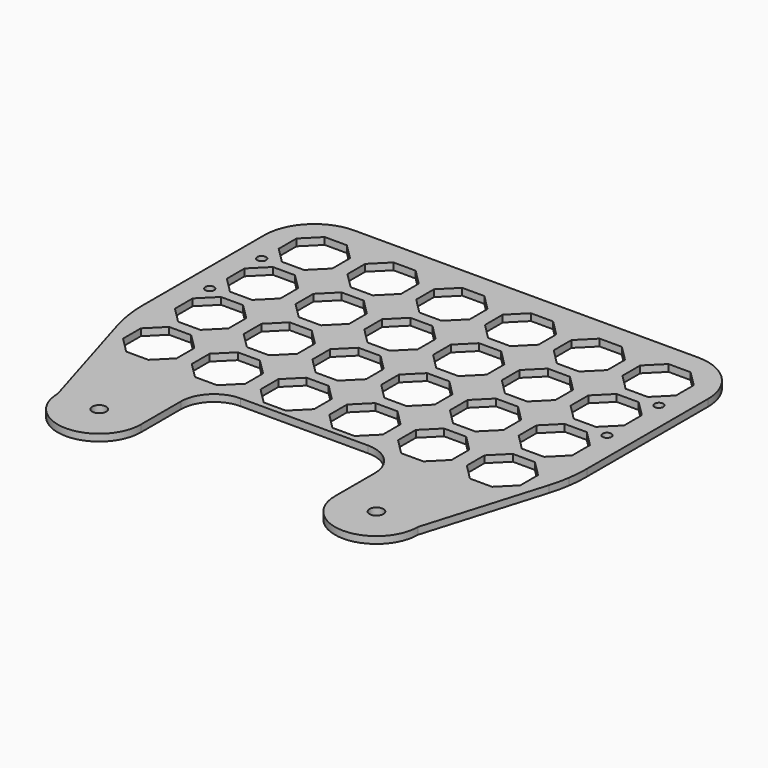
from build123d import *

# Parameters (mm, degrees)
F1_DEPTH = 3.175
F2_R     = 2.032
F3_DEPTH = 3.176


with BuildPart() as f1:
    # F0 (on Top) → F1 (new body)
    with BuildSketch(Plane.XY):
        with BuildLine():
            ThreePointArc((108.9422454268, -59.7267696282), (110.0983598091, -55.2992659283), (110.9326233067, -50.8))
            Line((110.9326233067, -50.8), (-90.8920706761, -50.8))
            ThreePointArc((-90.8920706761, -50.8), (-90.0578071784, -55.2992659283), (-88.9016927962, -59.7267696282))
            Line((-88.9016927962, -59.7267696282), (-72.5297236847, -114.3))
            ThreePointArc((-72.5297236847, -114.3), (-53.4797236847, -95.25), (-34.4297236847, -114.3))
            Line((-34.4297236847, -114.3), (-34.4297236847, -91.44))
            ThreePointArc((-34.4297236847, -91.44), (-29.96603103, -80.6636926547), (-19.1897236847, -76.2))
            Line((-19.1897236847, -76.2), (39.2302763153, -76.2))
            ThreePointArc((39.2302763153, -76.2), (50.0065836606, -80.6636926547), (54.4702763153, -91.44))
            Line((54.4702763153, -91.44), (54.4702763153, -114.3))
            ThreePointArc((54.4702763153, -114.3), (73.5202763153, -95.25), (92.5702763153, -114.3))
            Line((92.5702763153, -114.3), (108.9422454268, -59.7267696282))
        make_face()
        with BuildLine():
            Line((-90.8920706761, -50.8), (110.9326233067, -50.8))
            ThreePointArc((110.9326233067, -50.8), (111.448129721, -46.1527566655), (111.6202763153, -41.4801788947))
            Line((111.6202763153, -41.4801788947), (111.6202763153, 27.94))
            ThreePointArc((111.6202763153, 27.94), (104.9247373332, 44.1044610179), (88.7602763153, 50.8))
            Line((88.7602763153, 50.8), (-68.7197236847, 50.8))
            ThreePointArc((-68.7197236847, 50.8), (-84.8841847026, 44.1044610179), (-91.5797236847, 27.94))
            Line((-91.5797236847, 27.94), (-91.5797236847, -41.4801788947))
            ThreePointArc((-91.5797236847, -41.4801788947), (-91.4075770904, -46.1527566655), (-90.8920706761, -50.8))
        make_face()
        with BuildLine():
            ThreePointArc((54.4702763153, -114.3), (73.5202763153, -133.35), (92.5702763153, -114.3))
            Line((92.5702763153, -114.3), (76.6952763153, -114.3))
            ThreePointArc((76.6952763153, -114.3), (73.5202763153, -117.475), (70.3452763153, -114.3))
            Line((70.3452763153, -114.3), (54.4702763153, -114.3))
        make_face()
        with BuildLine():
            Line((76.6952763153, -114.3), (92.5702763153, -114.3))
            ThreePointArc((92.5702763153, -114.3), (73.5202763153, -95.25), (54.4702763153, -114.3))
            Line((54.4702763153, -114.3), (70.3452763153, -114.3))
            ThreePointArc((70.3452763153, -114.3), (73.5202763153, -111.125), (76.6952763153, -114.3))
        make_face()
        with BuildLine():
            ThreePointArc((-34.4297236847, -114.3), (-53.4797236847, -95.25), (-72.5297236847, -114.3))
            Line((-72.5297236847, -114.3), (-56.6547236847, -114.3))
            ThreePointArc((-56.6547236847, -114.3), (-53.4797236847, -111.125), (-50.3047236847, -114.3))
            Line((-50.3047236847, -114.3), (-34.4297236847, -114.3))
        make_face()
        with BuildLine():
            Line((-56.6547236847, -114.3), (-72.5297236847, -114.3))
            ThreePointArc((-72.5297236847, -114.3), (-53.4797236847, -133.35), (-34.4297236847, -114.3))
            Line((-34.4297236847, -114.3), (-50.3047236847, -114.3))
            ThreePointArc((-50.3047236847, -114.3), (-53.4797236847, -117.475), (-56.6547236847, -114.3))
        make_face()
    extrude(amount=F1_DEPTH)

    # F2 (on face) → F3 (cut, through all)
    with BuildSketch(Plane.XY.offset(3.175)):
        Polygon((-63.6397236847, 40.2042048969), (-73.7997236847, 40.2042048969), (-80.9839285816, 33.02), (-80.9839285816, 22.86), (-73.7997236847, 15.6757951031), (-63.6397236847, 15.6757951031), (-56.4555187878, 22.86), (-56.4555187878, 33.02), align=None)
        Polygon((-73.7997236847, -14.0422048969), (-63.6397236847, -14.0422048969), (-56.4555187878, -6.858), (-56.4555187878, 3.302), (-63.6397236847, 10.4862048969), (-73.7997236847, 10.4862048969), (-80.9839285816, 3.302), (-80.9839285816, -6.858), align=None)
        Polygon((-73.7997236847, -43.7602048969), (-63.6397236847, -43.7602048969), (-56.4555187878, -36.576), (-56.4555187878, -26.416), (-63.6397236847, -19.2317951031), (-73.7997236847, -19.2317951031), (-80.9839285816, -26.416), (-80.9839285816, -36.576), align=None)
        Polygon((-73.7997236847, -73.4782048969), (-63.6397236847, -73.4782048969), (-56.4555187878, -66.294), (-56.4555187878, -56.134), (-63.6397236847, -48.9497951031), (-73.7997236847, -48.9497951031), (-80.9839285816, -56.134), (-80.9839285816, -66.294), align=None)
        Polygon((-42.3037236847, 15.6757951031), (-32.1437236847, 15.6757951031), (-24.9595187878, 22.86), (-24.9595187878, 33.02), (-32.1437236847, 40.2042048969), (-42.3037236847, 40.2042048969), (-49.4879285816, 33.02), (-49.4879285816, 22.86), align=None)
        Polygon((-42.3037236847, -14.0422048969), (-32.1437236847, -14.0422048969), (-24.9595187878, -6.858), (-24.9595187878, 3.302), (-32.1437236847, 10.4862048969), (-42.3037236847, 10.4862048969), (-49.4879285816, 3.302), (-49.4879285816, -6.858), align=None)
        Polygon((-42.3037236847, -43.7602048969), (-32.1437236847, -43.7602048969), (-24.9595187878, -36.576), (-24.9595187878, -26.416), (-32.1437236847, -19.2317951031), (-42.3037236847, -19.2317951031), (-49.4879285816, -26.416), (-49.4879285816, -36.576), align=None)
        Polygon((-42.3037236847, -73.4782048969), (-32.1437236847, -73.4782048969), (-24.9595187878, -66.294), (-24.9595187878, -56.134), (-32.1437236847, -48.9497951031), (-42.3037236847, -48.9497951031), (-49.4879285816, -56.134), (-49.4879285816, -66.294), align=None)
        Polygon((-10.8077236847, 15.6757951031), (-0.6477236847, 15.6757951031), (6.5364812122, 22.86), (6.5364812122, 33.02), (-0.6477236847, 40.2042048969), (-10.8077236847, 40.2042048969), (-17.9919285816, 33.02), (-17.9919285816, 22.86), align=None)
        Polygon((-10.8077236847, -14.0422048969), (-0.6477236847, -14.0422048969), (6.5364812122, -6.858), (6.5364812122, 3.302), (-0.6477236847, 10.4862048969), (-10.8077236847, 10.4862048969), (-17.9919285816, 3.302), (-17.9919285816, -6.858), align=None)
        Polygon((-10.8077236847, -43.7602048969), (-0.6477236847, -43.7602048969), (6.5364812122, -36.576), (6.5364812122, -26.416), (-0.6477236847, -19.2317951031), (-10.8077236847, -19.2317951031), (-17.9919285816, -26.416), (-17.9919285816, -36.576), align=None)
        Polygon((-10.8077236847, -73.4782048969), (-0.6477236847, -73.4782048969), (6.5364812122, -66.294), (6.5364812122, -56.134), (-0.6477236847, -48.9497951031), (-10.8077236847, -48.9497951031), (-17.9919285816, -56.134), (-17.9919285816, -66.294), align=None)
        Polygon((20.6882763153, 15.6757951031), (30.8482763153, 15.6757951031), (38.0324812122, 22.86), (38.0324812122, 33.02), (30.8482763153, 40.2042048969), (20.6882763153, 40.2042048969), (13.5040714184, 33.02), (13.5040714184, 22.86), align=None)
        Polygon((20.6882763153, -14.0422048969), (30.8482763153, -14.0422048969), (38.0324812122, -6.858), (38.0324812122, 3.302), (30.8482763153, 10.4862048969), (20.6882763153, 10.4862048969), (13.5040714184, 3.302), (13.5040714184, -6.858), align=None)
        Polygon((20.6882763153, -43.7602048969), (30.8482763153, -43.7602048969), (38.0324812122, -36.576), (38.0324812122, -26.416), (30.8482763153, -19.2317951031), (20.6882763153, -19.2317951031), (13.5040714184, -26.416), (13.5040714184, -36.576), align=None)
        Polygon((20.6882763153, -73.4782048969), (30.8482763153, -73.4782048969), (38.0324812122, -66.294), (38.0324812122, -56.134), (30.8482763153, -48.9497951031), (20.6882763153, -48.9497951031), (13.5040714184, -56.134), (13.5040714184, -66.294), align=None)
        Polygon((52.1842763153, 15.6757951031), (62.3442763153, 15.6757951031), (69.5284812122, 22.86), (69.5284812122, 33.02), (62.3442763153, 40.2042048969), (52.1842763153, 40.2042048969), (45.0000714184, 33.02), (45.0000714184, 22.86), align=None)
        Polygon((52.1842763153, -14.0422048969), (62.3442763153, -14.0422048969), (69.5284812122, -6.858), (69.5284812122, 3.302), (62.3442763153, 10.4862048969), (52.1842763153, 10.4862048969), (45.0000714184, 3.302), (45.0000714184, -6.858), align=None)
        Polygon((52.1842763153, -43.7602048969), (62.3442763153, -43.7602048969), (69.5284812122, -36.576), (69.5284812122, -26.416), (62.3442763153, -19.2317951031), (52.1842763153, -19.2317951031), (45.0000714184, -26.416), (45.0000714184, -36.576), align=None)
        Polygon((52.1842763153, -73.4782048969), (62.3442763153, -73.4782048969), (69.5284812122, -66.294), (69.5284812122, -56.134), (62.3442763153, -48.9497951031), (52.1842763153, -48.9497951031), (45.0000714184, -56.134), (45.0000714184, -66.294), align=None)
        Polygon((83.6802763153, 15.6757951031), (93.8402763153, 15.6757951031), (101.0244812122, 22.86), (101.0244812122, 33.02), (93.8402763153, 40.2042048969), (83.6802763153, 40.2042048969), (76.4960714184, 33.02), (76.4960714184, 22.86), align=None)
        Polygon((83.6802763153, -14.0422048969), (93.8402763153, -14.0422048969), (101.0244812122, -6.858), (101.0244812122, 3.302), (93.8402763153, 10.4862048969), (83.6802763153, 10.4862048969), (76.4960714184, 3.302), (76.4960714184, -6.858), align=None)
        Polygon((83.6802763153, -43.7602048969), (93.8402763153, -43.7602048969), (101.0244812122, -36.576), (101.0244812122, -26.416), (93.8402763153, -19.2317951031), (83.6802763153, -19.2317951031), (76.4960714184, -26.416), (76.4960714184, -36.576), align=None)
        Polygon((83.6802763153, -73.4782048969), (93.8402763153, -73.4782048969), (101.0244812122, -66.294), (101.0244812122, -56.134), (93.8402763153, -48.9497951031), (83.6802763153, -48.9497951031), (76.4960714184, -56.134), (76.4960714184, -66.294), align=None)
        with Locations((-80.9839285816, 13.081)):
            Circle(F2_R)
        with Locations((-80.9839285816, -16.637)):
            Circle(F2_R)
        with Locations((101.0244812122, 13.081)):
            Circle(F2_R)
        with Locations((101.0244812122, -16.637)):
            Circle(F2_R)
    extrude(amount=-F3_DEPTH, mode=Mode.SUBTRACT)


solid = f1.part
